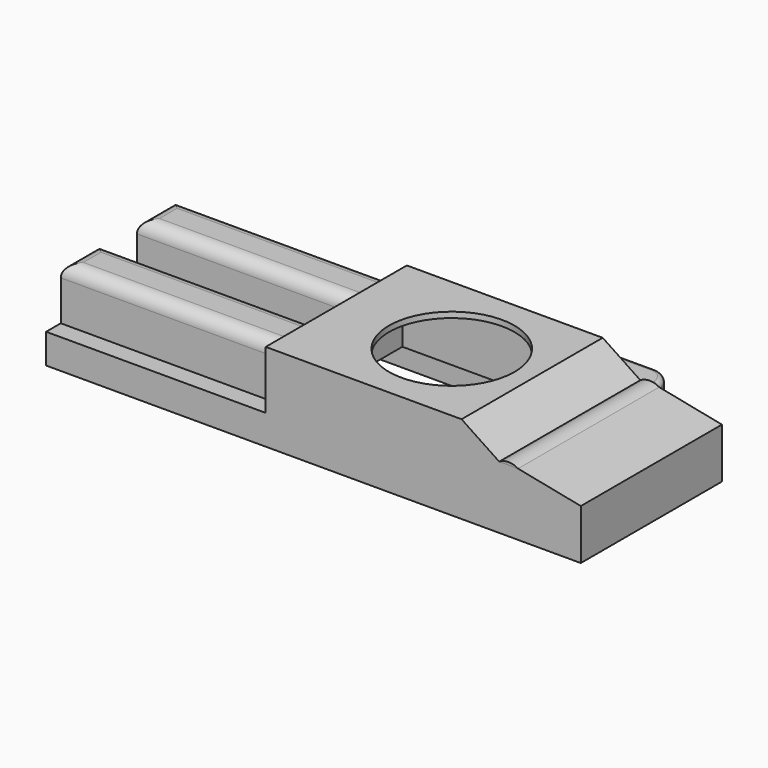
from build123d import *

# Parameters (mm, degrees)
F0_W        = 94.5233479142
F0_H        = 71.4051574469
F1_DEPTH    = 35.56
F2_R        = 25.4
F3_DEPTH    = 35.56
F4_SIZE2    = 15.24
F4_SIZE     = 10.16
F5_DEPTH    = 7.62
F7_DEPTH    = 71.4051658
F8_DEPTH    = 25.4
F9_T4_DEPTH = 203.3902674307
F9_S5_R     = 7.295449901
F9_T6_DEPTH = 104
F10_W       = 71.4051574469
F10_H       = 12.0417065918
F11_DEPTH   = 88.9
F12_W       = 19.05
F12_H       = 21.2708730352
F13_DEPTH   = 88.9
F14_W       = 19.05
F14_H       = 21.2708730352
F15_DEPTH   = 88.9
F16_R       = 5.08
F17_W       = 97.8622660041
F17_H       = 11.2377274781
F18_DEPTH   = 12.7
F19_R       = 7.62
F20_R       = 2.032
F21_W       = 212.6409783959
F21_H       = 67.3823393881
F22_DEPTH   = 8.89
F23_W       = 78.3353857696
F23_H       = 65.2360282838
F24_DEPTH   = 24.384


# Not quite as in the source:
# - a fillet or chamfer that OpenCascade refuses, or shapes differently, is made with other operations: its cross-section is extruded or revolved along the edge and cut away or added


with BuildPart() as f1:
    # F0 (on Top) → F1 (new body)
    with BuildSketch(Plane.XY):
        with Locations((0.5442798138, -0.0245943666)):
            Rectangle(F0_W, F0_H)
    extrude(amount=F1_DEPTH)

    # F2 (on Top) → F3 (cut)
    with BuildSketch(Plane.XY):
        Circle(F2_R)
    extrude(amount=F3_DEPTH, mode=Mode.SUBTRACT)

    # F4
    f4_edges = [f1.edges().sort_by_distance(p)[0] for p in [
        (47.805954, -0.024594, 35.56),
    ]]
    f4_side = f1.faces().sort_by_distance((47.805954, -0.024594, 17.78))[0]
    chamfer(f4_edges, length=F4_SIZE, length2=F4_SIZE2, reference=f4_side)

    # F5 (add): a face of the model
    f5_faces = [f1.faces().sort_by_distance(p)[0] for p in [
        (47.8059537709, -0.0245943666, 12.7),
    ]]
    extrude(f5_faces, amount=F5_DEPTH)

    # F6 (on face) → F7 (join)
    with BuildSketch(Plane(origin=(0, 35.6779843569, 0), x_dir=(-1, 0, 0), z_dir=(0, 1, 0))):
        with BuildLine():
            Line((-55.4259537709, 25.4), (-47.8059537709, 25.4))
            ThreePointArc((-47.8059537709, 25.4), (-51.6159537709, 26.473915584), (-55.4259537709, 25.4))
        make_face()
    extrude(amount=-F7_DEPTH)

    # F8 (add): a face of the model
    f8_faces = [f1.faces().sort_by_distance(p)[0] for p in [
        (55.4259537709, -0.0245943666, 12.7),
    ]]
    extrude(f8_faces, amount=F8_DEPTH)

    # F9: chamfer of 5.08 x 25.4 on 1 edges, made by hand


with BuildPart() as f9_tool2:
    # F9_s3 → F9_t4 (new body)
    with BuildSketch(Plane.XZ.offset(101.7197280819)):
        Polygon((55.4259537709, 25.4), (80.8259537709, 20.32), (80.8259537709, 25.4), align=None)
    extrude(amount=-F9_T4_DEPTH)

    # F9_s5 → F9_t6 (cut, symmetric)
    with BuildSketch(Plane.XZ):
        with Locations((51.6159537709, 19.178465683)):
            Circle(F9_S5_R)
    extrude(amount=F9_T6_DEPTH, both=True, mode=Mode.SUBTRACT)


with BuildPart() as f1_1:
    add(f1.part)

    # F9_t1: cut F9_tool2
    add(f9_tool2.part, mode=Mode.SUBTRACT)

    # F10 (on face) → F11 (join)
    with BuildSketch(Plane(origin=(-46.7173941433, 0, 0), x_dir=(0, -1, 0), z_dir=(-1, 0, 0))):
        with Locations((0.0245943666, 6.0208532959)):
            Rectangle(F10_W, F10_H)
    extrude(amount=F11_DEPTH)

    # F12 (on face) → F13 (join)
    with BuildSketch(Plane(origin=(-46.7173941433, 0, 0), x_dir=(0, -1, 0), z_dir=(-1, 0, 0))):
        with Locations((-19.7377734572, 22.6771431095)):
            Rectangle(F12_W, F12_H)
    extrude(amount=F13_DEPTH)

    # F14 (on face) → F15 (join)
    with BuildSketch(Plane(origin=(-46.7173941433, 0, 0), x_dir=(0, -1, 0), z_dir=(-1, 0, 0))):
        with Locations((18.7768059537, 22.6771431095)):
            Rectangle(F14_W, F14_H)
    extrude(amount=F15_DEPTH)

    # F16
    f16_edges = [f1_1.edges().sort_by_distance(p)[0] for p in [
        (-91.167394, 29.262773, 33.31258),
        (-91.167394, 10.212773, 33.31258),
        (-91.167394, -9.251806, 33.31258),
        (-91.167394, -28.301806, 33.31258),
        (-135.617394, 19.737773, 33.31258),
        (-135.617394, -18.776806, 33.31258),
    ]]
    fillet(f16_edges, radius=F16_R)

    # F17 (on face) → F18 (join)
    with BuildSketch(Plane(origin=(0, 35.6779843569, 0), x_dir=(-1, 0, 0), z_dir=(0, 1, 0))):
        with Locations((-2.2137388587, 17.6605703309)):
            Rectangle(F17_W, F17_H)
    extrude(amount=F18_DEPTH)

    # F19
    f19_edges = [f1_1.edges().sort_by_distance(p)[0] for p in [
        (51.144872, 48.377984, 17.66057),
    ]]
    fillet(f19_edges, radius=F19_R)

    # F20
    f20_edges = [f1_1.edges().sort_by_distance(p)[0] for p in [
        (48.913026, 46.146138, 23.279434),
        (51.144872, 38.217984, 23.279434),
        (-1.596261, 48.377984, 23.279434),
        (51.144872, 38.217984, 12.041707),
        (48.913026, 46.146138, 12.041707),
        (-1.596261, 48.377984, 12.041707),
    ]]
    fillet(f20_edges, radius=F20_R)

    # F21 (on face) → F22 (cut, symmetric)
    with BuildSketch(Plane(origin=(0, 0, 0), x_dir=(1, 0, 0), z_dir=(0, 0, -1))):
        with Locations((-27.7419649065, 0.2171527594)):
            Rectangle(F21_W, F21_H)
    extrude(amount=F22_DEPTH, both=True, mode=Mode.SUBTRACT)

    # F23 (on face) → F24 (cut)
    with BuildSketch(Plane(origin=(0, 0, 8.89), x_dir=(1, 0, 0), z_dir=(0, 0, -1))):
        with Locations((-5.8767069131, 1.2903083116)):
            Rectangle(F23_W, F23_H)
    extrude(amount=-F24_DEPTH, mode=Mode.SUBTRACT)


solid = f1_1.part
